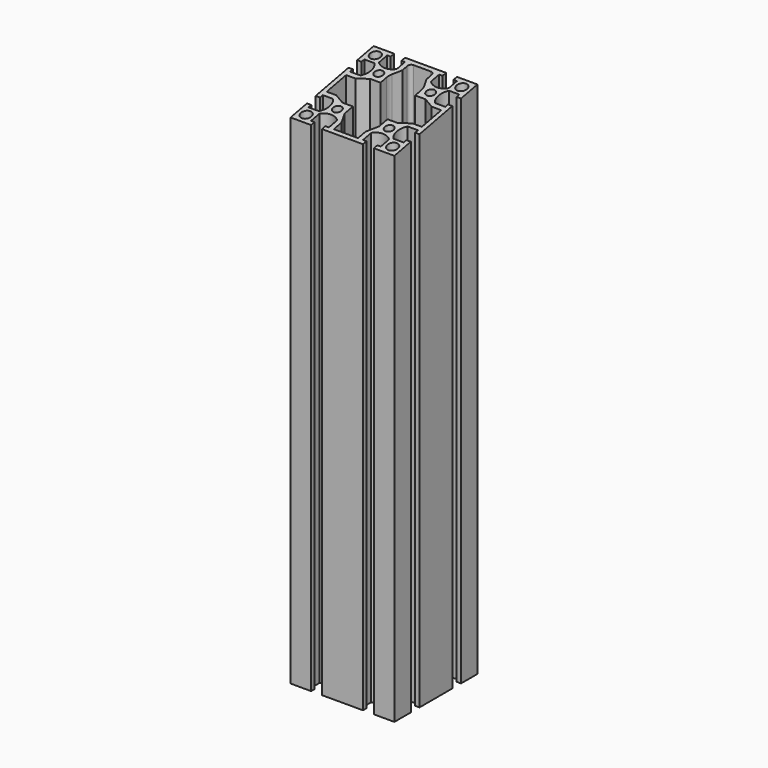
from build123d import *

# Parameters (mm, degrees)
F0_R          = 3
F0_R_2        = 2.5
F1_DEPTH      = 300
F2_R          = 2
F3_R          = 7
F5_DEPTH      = 30
F5_DEPTH_BACK = 30


# Not quite as in the source:
# - a feature names something its author has since deleted; it is built from what else it names


with BuildPart() as f1:
    # F0 (on Top) → F1 (new body)
    with BuildSketch(Plane.XY):
        with BuildLine():
            Line((18.15, -30), (30, -30))
            Line((30, -30), (30, -18.15))
            Line((30, -18.15), (27.5, -18.15))
            Line((27.5, -18.15), (27.5, -20.15))
            Line((27.5, -20.15), (21.5477069044, -20.15))
            ThreePointArc((21.5477069044, -20.15), (19.5, -15), (21.5477069044, -9.85))
            Line((21.5477069044, -9.85), (27.5, -9.85))
            Line((27.5, -9.85), (27.5, -11.85))
            Line((27.5, -11.85), (30, -11.85))
            Line((30, -11.85), (30, 11.85))
            Line((30, 11.85), (27.5, 11.85))
            Line((27.5, 11.85), (27.5, 9.85))
            Line((27.5, 9.85), (21.5477069044, 9.85))
            ThreePointArc((21.5477069044, 9.85), (19.5, 15), (21.5477069044, 20.15))
            Line((21.5477069044, 20.15), (27.5, 20.15))
            Line((27.5, 20.15), (27.5, 18.15))
            Line((27.5, 18.15), (30, 18.15))
            Line((30, 18.15), (30, 30))
            Line((30, 30), (18.15, 30))
            Line((18.15, 30), (18.15, 27.5))
            Line((18.15, 27.5), (20.15, 27.5))
            Line((20.15, 27.5), (20.15, 21.5477069044))
            ThreePointArc((20.15, 21.5477069044), (15, 19.5), (9.85, 21.5477069044))
            Line((9.85, 21.5477069044), (9.85, 27.5))
            Line((9.85, 27.5), (11.85, 27.5))
            Line((11.85, 27.5), (11.85, 30))
            Line((11.85, 30), (-11.85, 30))
            Line((-11.85, 30), (-11.85, 27.5))
            Line((-11.85, 27.5), (-9.85, 27.5))
            Line((-9.85, 27.5), (-9.85, 21.5477069044))
            ThreePointArc((-9.85, 21.5477069044), (-15, 19.5), (-20.15, 21.5477069044))
            Line((-20.15, 21.5477069044), (-20.15, 27.5))
            Line((-20.15, 27.5), (-18.15, 27.5))
            Line((-18.15, 27.5), (-18.15, 30))
            Line((-18.15, 30), (-30, 30))
            Line((-30, 30), (-30, 18.15))
            Line((-30, 18.15), (-27.5, 18.15))
            Line((-27.5, 18.15), (-27.5, 20.15))
            Line((-27.5, 20.15), (-21.5477069044, 20.15))
            ThreePointArc((-21.5477069044, 20.15), (-19.5, 15), (-21.5477069044, 9.85))
            Line((-21.5477069044, 9.85), (-27.5, 9.85))
            Line((-27.5, 9.85), (-27.5, 11.85))
            Line((-27.5, 11.85), (-30, 11.85))
            Line((-30, 11.85), (-30, -11.85))
            Line((-30, -11.85), (-27.5, -11.85))
            Line((-27.5, -11.85), (-27.5, -9.85))
            Line((-27.5, -9.85), (-21.5477069044, -9.85))
            ThreePointArc((-21.5477069044, -9.85), (-19.5, -15), (-21.5477069044, -20.15))
            Line((-21.5477069044, -20.15), (-27.5, -20.15))
            Line((-27.5, -20.15), (-27.5, -18.15))
            Line((-27.5, -18.15), (-30, -18.15))
            Line((-30, -18.15), (-30, -30))
            Line((-30, -30), (-18.15, -30))
            Line((-18.15, -30), (-18.15, -27.5))
            Line((-18.15, -27.5), (-20.15, -27.5))
            Line((-20.15, -27.5), (-20.15, -21.5477069044))
            ThreePointArc((-20.15, -21.5477069044), (-15, -19.5), (-9.85, -21.5477069044))
            Line((-9.85, -21.5477069044), (-9.85, -27.5))
            Line((-9.85, -27.5), (-11.85, -27.5))
            Line((-11.85, -27.5), (-11.85, -30))
            Line((-11.85, -30), (11.85, -30))
            Line((11.85, -30), (11.85, -27.5))
            Line((11.85, -27.5), (9.85, -27.5))
            Line((9.85, -27.5), (9.85, -21.5477069044))
            ThreePointArc((9.85, -21.5477069044), (15, -19.5), (20.15, -21.5477069044))
            Line((20.15, -21.5477069044), (20.15, -27.5))
            Line((20.15, -27.5), (18.15, -27.5))
            Line((18.15, -27.5), (18.15, -30))
        make_face()
        with Locations((-25, -25)):
            Circle(F0_R, mode=Mode.SUBTRACT)
        with Locations((-15, -15)):
            Circle(F0_R_2, mode=Mode.SUBTRACT)
        with Locations((25, -25)):
            Circle(F0_R, mode=Mode.SUBTRACT)
        with Locations((15, -15)):
            Circle(F0_R_2, mode=Mode.SUBTRACT)
        with Locations((-25, 25)):
            Circle(F0_R, mode=Mode.SUBTRACT)
        with Locations((-15, 15)):
            Circle(F0_R_2, mode=Mode.SUBTRACT)
        Polygon((-7, 22), (-7, 27.5), (0, 27.5), (7, 27.5), (7, 22), (10, 16), (10, 10), (16, 10), (22, 7), (27.5, 7), (27.5, 0), (27.5, -7), (22, -7), (16, -10), (10, -10), (10, -16), (7, -22), (7, -27.5), (0, -27.5), (-7, -27.5), (-7, -22), (-10, -16), (-10, -10), (-16, -10), (-22, -7), (-27.5, -7), (-27.5, 0), (-27.5, 7), (-22, 7), (-16, 10), (-10, 10), (-10, 16), align=None, mode=Mode.SUBTRACT)
        with Locations((15, 15)):
            Circle(F0_R_2, mode=Mode.SUBTRACT)
        with Locations((25, 25)):
            Circle(F0_R, mode=Mode.SUBTRACT)
    extrude(amount=F1_DEPTH)

    # F2
    f2_edges = [f1.edges().sort_by_distance(p)[0] for p in [
        (-7, 27.5, 150),
        (7, 27.5, 150),
    ]]
    fillet(f2_edges, radius=F2_R)

    # F3
    f3_edges = [f1.edges().sort_by_distance(p)[0] for p in [
        (-10, 16, 150),
        (10, 16, 150),
    ]]
    fillet(f3_edges, radius=F3_R)

    # F4 (on Right) → F5 (cut, two sides)
    with BuildSketch(Plane.YZ) as f5_sk:
        Polygon((-20.5082305996, 553.922022371), (-199.5184071674, 518.3146843648), (-149.0101765678, 264.3926619939), (30, 300), align=None)
    extrude(amount=F5_DEPTH, mode=Mode.SUBTRACT)
    extrude(f5_sk.sketch, amount=-F5_DEPTH_BACK, mode=Mode.SUBTRACT)


solid = f1.part
